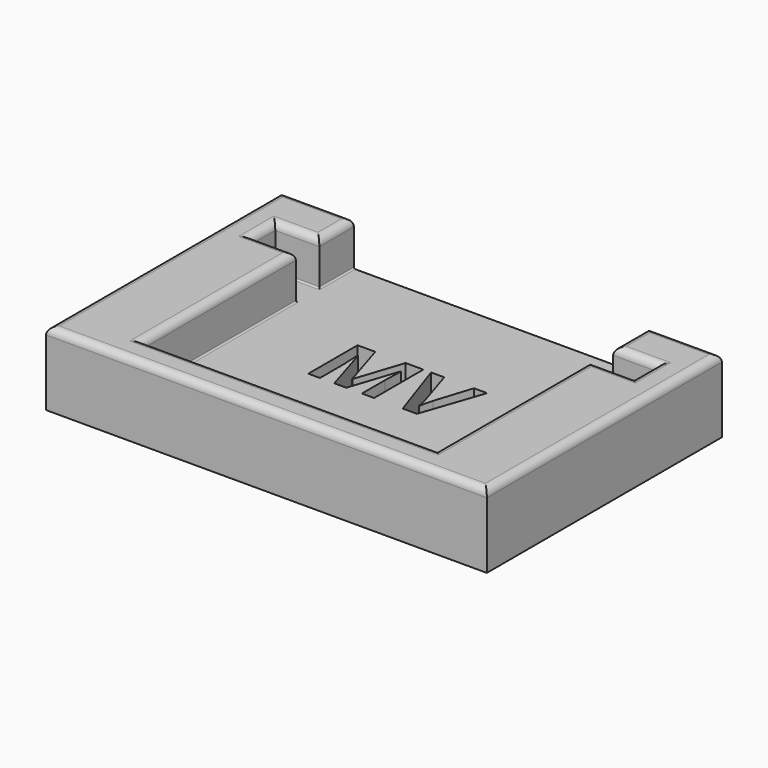
from build123d import *

# Parameters (mm, degrees)
F1_DEPTH     = 3
F3_DEPTH     = 2
F4_R         = 0.5
F5_R         = 0.1
F6_TEXT_SIZE = 5.870024001
F7_DEPTH     = 2.001


# Not quite as in the source:
# - Text() gives the source's letters only with a copy of the font that has no kerning and outlines rounded to 1/6400 em; it was checked with that copy


with BuildPart() as f1:
    # F0 (on Top) → F1 (new body)
    with BuildSketch(Plane.XY):
        Polygon((5, 20), (0, 20), (0, 0), (30, 0), (30, 20), (25, 20), (25, 17), (28, 17), (28, 15), (25, 15), (25, 2), (5, 2), (5, 15), (2, 15), (2, 17), (5, 17), align=None)
    extrude(amount=F1_DEPTH)

    # F2 (on face) → F3 (join)
    with BuildSketch(Plane(origin=(0, 0, 0), x_dir=(1, 0, 0), z_dir=(0, 0, -1))):
        Polygon((5, -17), (5, -20), (25, -20), (25, -17), (28, -17), (28, -15), (25, -15), (25, -2), (5, -2), (5, -15), (2, -15), (2, -17), align=None)
        Polygon((30, 0), (0, 0), (0, -20), (5, -20), (5, -17), (2, -17), (2, -15), (5, -15), (5, -2), (25, -2), (25, -15), (28, -15), (28, -17), (25, -17), (25, -20), (30, -20), align=None)
    extrude(amount=F3_DEPTH)

    # F4
    f4_edges = [f1.edges().sort_by_distance(p)[0] for p in [
        (2.5, 20, 3),
        (0, 10, 3),
        (15, 0, 3),
        (30, 10, 3),
        (27.5, 20, 3),
        (25, 18.5, 3),
        (26.5, 17, 3),
        (28, 16, 3),
        (26.5, 15, 3),
        (25, 8.5, 3),
        (15, 2, 3),
        (5, 8.5, 3),
        (3.5, 15, 3),
        (2, 16, 3),
        (3.5, 17, 3),
        (5, 18.5, 3),
    ]]
    fillet(f4_edges, radius=F4_R)

    # F5
    f5_edges = [f1.edges().sort_by_distance(p)[0] for p in [
        (15, 20, 0),
        (5, 18.5, 0),
        (3.5, 17, 0),
        (2, 16, 0),
        (3.5, 15, 0),
        (5, 8.5, 0),
        (15, 2, 0),
        (25, 8.5, 0),
        (26.5, 15, 0),
        (28, 16, 0),
        (26.5, 17, 0),
        (25, 18.5, 0),
        (5, 20, 1.25),
        (25, 20, 1.25),
        (4.853553, 19.853553, 2.853553),
        (25.146447, 19.853553, 2.853553),
    ]]
    fillet(f5_edges, radius=F5_R)

    # F6 (on face) → F7 (cut, through all)
    with BuildSketch(Plane.XY):
        with Locations((10.1352176092, 8.9784460142)):
            Text('MV', F6_TEXT_SIZE, font='Open Sans', font_style=FontStyle.BOLD, text_align=(TextAlign.LEFT, TextAlign.BOTTOM))
    extrude(amount=-F7_DEPTH, mode=Mode.SUBTRACT)


solid = f1.part
